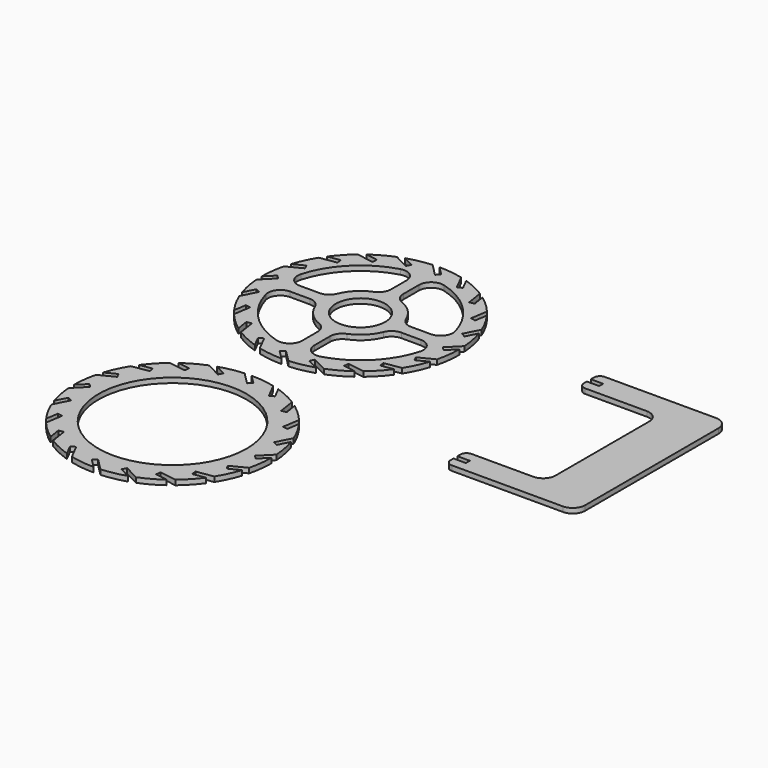
from build123d import *

# Parameters (mm, degrees)
F0_R     = 20
F1_DEPTH = 4
F0_R_2   = 60


# Not quite as in the source:
# - ends of sketch curves that miss each other by under 0.0002 mm in the source are joined


with BuildPart() as f1:
    # F0 (on Top) → F1 (new body)
    with BuildSketch(Plane.XY):
        with BuildLine():
            ThreePointArc((-98.2949099027, 172.7183773881), (-107.951775958, 174.5185802967), (-117.756472, 175.121679))
            Line((-117.756472, 175.121679), (-110.685404, 168.050611))
            Line((-110.685404, 168.050611), (-113.513831, 165.222184))
            Line((-113.513831, 165.222184), (-123.226125, 174.934478))
            ThreePointArc((-123.226125, 174.934478), (-132.9666439698, 173.6624370091), (-142.4778320463, 171.2062001424))
            Line((-142.4778320463, 171.2062001424), (-133.567766, 166.666295))
            Line((-133.567766, 166.666295), (-135.383728, 163.102269))
            Line((-135.383728, 163.102269), (-147.621933, 169.337946))
            ThreePointArc((-147.621933, 169.337946), (-156.4926341286, 165.1181769356), (-164.779292, 159.843038))
            Line((-164.779292, 159.843038), (-154.902409, 158.278694))
            Line((-154.902409, 158.278694), (-155.528147, 154.32794))
            Line((-155.528147, 154.32794), (-169.094301, 156.476608))
            ThreePointArc((-169.094301, 156.476608), (-176.2268590711, 149.7221719992), (-182.4778317927, 142.1444988494))
            Line((-182.4778317927, 142.1444988494), (-172.600948, 143.708844))
            Line((-172.600948, 143.708844), (-171.97521, 139.75809))
            Line((-171.97521, 139.75809), (-185.541364, 137.609423))
            ThreePointArc((-185.541364, 137.609423), (-190.2375947091, 128.9814907365), (-193.8409934363, 119.8430381417))
            Line((-193.8409934363, 119.8430381417), (-184.930928, 124.382943))
            Line((-184.930928, 124.382943), (-183.114966, 120.818917))
            Line((-183.114966, 120.818917), (-195.35317, 114.583241))
            ThreePointArc((-195.35317, 114.583241), (-197.1533732967, 104.926375042), (-197.756472, 95.121679))
            Line((-197.756472, 95.121679), (-190.685404, 102.192747))
            Line((-190.685404, 102.192747), (-187.856977, 99.36432))
            Line((-187.856977, 99.36432), (-197.569271, 89.652026))
            ThreePointArc((-197.569271, 89.652026), (-196.2972300091, 79.9115070302), (-193.8409931424, 70.4003189537))
            Line((-193.8409931424, 70.4003189537), (-189.301088, 79.310385))
            Line((-189.301088, 79.310385), (-185.737062, 77.494423))
            Line((-185.737062, 77.494423), (-191.972739, 65.256218))
            ThreePointArc((-191.972739, 65.256218), (-187.7529701762, 56.3855170442), (-182.4778317927, 48.0988591506))
            Line((-182.4778317927, 48.0988591506), (-180.913487, 57.975742))
            Line((-180.913487, 57.975742), (-176.962734, 57.350004))
            Line((-176.962734, 57.350004), (-179.111401, 43.78385))
            ThreePointArc((-179.111401, 43.78385), (-172.3569649992, 36.6512919289), (-164.7792918494, 30.4003192073))
            Line((-164.7792918494, 30.4003192073), (-166.343637, 40.277203))
            Line((-166.343637, 40.277203), (-162.392883, 40.902941))
            Line((-162.392883, 40.902941), (-160.244216, 27.336787))
            ThreePointArc((-160.244216, 27.336787), (-151.6162841674, 22.6405564922), (-142.4778320463, 19.0371578576))
            Line((-142.4778320463, 19.0371578576), (-147.017737, 27.947223))
            Line((-147.017737, 27.947223), (-143.45371, 29.763185))
            Line((-143.45371, 29.763185), (-137.218034, 17.52498))
            ThreePointArc((-137.218034, 17.52498), (-127.5611679213, 15.7247776884), (-117.756472, 15.121679))
            Line((-117.756472, 15.121679), (-124.82754, 22.192747))
            Line((-124.82754, 22.192747), (-121.999113, 25.021174))
            Line((-121.999113, 25.021174), (-112.286819, 15.30888))
            ThreePointArc((-112.286819, 15.30888), (-102.5463000302, 16.5809209909), (-93.0351119537, 19.0371578576))
            Line((-93.0351119537, 19.0371578576), (-101.945178, 23.577063))
            Line((-101.945178, 23.577063), (-100.129216, 27.141089))
            Line((-100.129216, 27.141089), (-87.891011, 20.905412))
            ThreePointArc((-87.891011, 20.905412), (-79.0203100442, 25.1251808238), (-70.7336521506, 30.4003192073))
            Line((-70.7336521506, 30.4003192073), (-80.610535, 31.964664))
            Line((-80.610535, 31.964664), (-79.984797, 35.915417))
            Line((-79.984797, 35.915417), (-66.418643, 33.76675))
            ThreePointArc((-66.418643, 33.76675), (-59.2860849289, 40.5211860008), (-53.0351122073, 48.0988591506))
            Line((-53.0351122073, 48.0988591506), (-62.911996, 46.534514))
            Line((-62.911996, 46.534514), (-63.537734, 50.485267))
            Line((-63.537734, 50.485267), (-49.97158, 52.633935))
            ThreePointArc((-49.97158, 52.633935), (-45.2753494922, 61.2618668326), (-41.6719508576, 70.4003189537))
            Line((-41.6719508576, 70.4003189537), (-50.582016, 65.860414))
            Line((-50.582016, 65.860414), (-52.397978, 69.42444))
            Line((-52.397978, 69.42444), (-40.159774, 75.660117))
            ThreePointArc((-40.159774, 75.660117), (-38.3595707033, 85.316982958), (-37.756472, 95.121679))
            Line((-37.756472, 95.121679), (-44.82754, 88.050611))
            Line((-44.82754, 88.050611), (-47.655967, 90.879038))
            Line((-47.655967, 90.879038), (-37.943673, 100.591332))
            ThreePointArc((-37.943673, 100.591332), (-39.2157139005, 110.3318505029), (-41.6719505637, 119.8430381417))
            Line((-41.6719505637, 119.8430381417), (-46.211856, 110.932973))
            Line((-46.211856, 110.932973), (-49.775882, 112.748935))
            Line((-49.775882, 112.748935), (-43.540205, 124.98714))
            ThreePointArc((-43.540205, 124.98714), (-47.7599738238, 133.8578409558), (-53.0351122073, 142.1444988494))
            Line((-53.0351122073, 142.1444988494), (-54.599457, 132.267616))
            Line((-54.599457, 132.267616), (-58.55021, 132.893354))
            Line((-58.55021, 132.893354), (-56.401543, 146.459508))
            ThreePointArc((-56.401543, 146.459508), (-63.155978786, 153.5920658705), (-70.7336516751, 159.8430384472))
            Line((-70.7336516751, 159.8430384472), (-69.169307, 149.966155))
            Line((-69.169307, 149.966155), (-73.120061, 149.340417))
            Line((-73.120061, 149.340417), (-75.268728, 162.906571))
            ThreePointArc((-75.268728, 162.906571), (-83.8966598326, 167.6028015078), (-93.0351119537, 171.2062001424))
            Line((-93.0351119537, 171.2062001424), (-88.495207, 162.296135))
            Line((-88.495207, 162.296135), (-92.059234, 160.480173))
            Line((-92.059234, 160.480173), (-98.2949099027, 172.7183773881))
        make_face()
        with BuildLine():
            Line((-170.673856, 90.129798), (-154.840804, 90.129798))
            ThreePointArc((-154.840804, 90.129798), (-149.2497262903, 88.420747888), (-145.5697349779, 83.8777680089))
            ThreePointArc((-145.5697349779, 83.8777680089), (-138.9697319753, 73.9084751041), (-129.0004390268, 67.3084719338))
            ThreePointArc((-129.0004390268, 67.3084719338), (-124.4574598529, 63.6284803253), (-122.74841, 58.037403))
            Line((-122.74841, 58.037403), (-122.74841, 42.204352))
            ThreePointArc((-122.74841, 42.204352), (-126.7175709587, 34.2275744265), (-135.4742060915, 32.5830196771))
            ThreePointArc((-135.4742060915, 32.5830196771), (-163.718469437, 49.1597378827), (-180.2951881241, 77.4040009648))
            ThreePointArc((-180.2951881241, 77.4040009648), (-178.6506338636, 86.1606366576), (-170.673856, 90.129798))
        make_face(mode=Mode.SUBTRACT)
        with BuildLine():
            Line((-112.764647, 42.204352), (-112.764647, 58.037403))
            ThreePointArc((-112.764647, 58.037403), (-111.0555971471, 63.6284803253), (-106.5126178685, 67.3084716746))
            ThreePointArc((-106.5126178685, 67.3084716746), (-96.5433255644, 73.9084755644), (-89.9433222812, 83.8777681137))
            ThreePointArc((-89.9433222812, 83.8777681137), (-86.2633307097, 88.420747888), (-80.672253, 90.129798))
            Line((-80.672253, 90.129798), (-64.839202, 90.129798))
            ThreePointArc((-64.839202, 90.129798), (-56.8624242186, 86.1606367663), (-55.2178698651, 77.4040012451))
            ThreePointArc((-55.2178698651, 77.4040012451), (-71.7945881265, 49.1597383192), (-100.0388509648, 32.5830198759))
            ThreePointArc((-100.0388509648, 32.5830198759), (-108.7954860413, 34.2275744265), (-112.764647, 42.204352))
        make_face(mode=Mode.SUBTRACT)
        with Locations((-117.756529, 95.121679)):
            Circle(F0_R, mode=Mode.SUBTRACT)
        with BuildLine():
            ThreePointArc((-145.5697349779, 106.3655899911), (-149.2497262903, 101.822610112), (-154.840804, 100.11356))
            Line((-154.840804, 100.11356), (-170.673856, 100.11356))
            ThreePointArc((-170.673856, 100.11356), (-178.6506338636, 104.0827213424), (-180.2951880606, 112.8393570172))
            ThreePointArc((-180.2951880606, 112.8393570172), (-163.718469437, 141.0836201173), (-135.4742061095, 157.6603383864))
            ThreePointArc((-135.4742061095, 157.6603383864), (-126.7175709587, 156.0157835735), (-122.74841, 148.039006))
            Line((-122.74841, 148.039006), (-122.74841, 132.205954))
            ThreePointArc((-122.74841, 132.205954), (-124.4574597481, 126.61487683), (-129.0004387841, 122.9348854659))
            ThreePointArc((-129.0004387841, 122.9348854659), (-138.9697319753, 116.3348828959), (-145.5697349779, 106.3655899911))
        make_face(mode=Mode.SUBTRACT)
        with BuildLine():
            Line((-64.839202, 100.11356), (-80.672253, 100.11356))
            ThreePointArc((-80.672253, 100.11356), (-86.2633307097, 101.822610112), (-89.9433220221, 106.3655899911))
            ThreePointArc((-89.9433220221, 106.3655899911), (-96.5433255644, 116.3348824356), (-106.5126181137, 122.9348857188))
            ThreePointArc((-106.5126181137, 122.9348857188), (-111.0555972519, 126.61487683), (-112.764647, 132.205954))
            Line((-112.764647, 132.205954), (-112.764647, 148.039006))
            ThreePointArc((-112.764647, 148.039006), (-108.7954860413, 156.0157835735), (-100.0388509085, 157.6603383229))
            ThreePointArc((-100.0388509085, 157.6603383229), (-71.7945881265, 141.0836196808), (-55.2178698016, 112.8393567729))
            ThreePointArc((-55.2178698016, 112.8393567729), (-56.8624242186, 104.0827212337), (-64.839202, 100.11356))
        make_face(mode=Mode.SUBTRACT)
    extrude(amount=F1_DEPTH)


with BuildPart() as f1b:
    # F0 (on Top) → F1, piece 2 (new body)
    with BuildSketch(Plane.XY):
        with BuildLine():
            ThreePointArc((-98.2949099027, -17.5249796119), (-107.951775958, -15.7247767033), (-117.756472, -15.121678))
            Line((-117.756472, -15.121678), (-110.685404, -22.192746))
            Line((-110.685404, -22.192746), (-113.513831, -25.021173))
            Line((-113.513831, -25.021173), (-123.226125, -15.308879))
            ThreePointArc((-123.226125, -15.308879), (-132.9666439698, -16.5809199909), (-142.4778320463, -19.0371568576))
            Line((-142.4778320463, -19.0371568576), (-133.567766, -23.577062))
            Line((-133.567766, -23.577062), (-135.383728, -27.141088))
            Line((-135.383728, -27.141088), (-147.621933, -20.905411))
            ThreePointArc((-147.621933, -20.905411), (-156.4926340905, -25.1251795775), (-164.779292, -30.400318))
            Line((-164.779292, -30.400318), (-154.902409, -31.964663))
            Line((-154.902409, -31.964663), (-155.528147, -35.915416))
            Line((-155.528147, -35.915416), (-169.094301, -33.766749))
            ThreePointArc((-169.094301, -33.766749), (-176.2268590711, -40.5211850008), (-182.4778317927, -48.0988581506))
            Line((-182.4778317927, -48.0988581506), (-172.600948, -46.534513))
            Line((-172.600948, -46.534513), (-171.97521, -50.485267))
            Line((-171.97521, -50.485267), (-185.541364, -52.633934))
            ThreePointArc((-185.541364, -52.633934), (-190.2375945078, -61.2618658326), (-193.8409931424, -70.4003179537))
            Line((-193.8409931424, -70.4003179537), (-184.930928, -65.860413))
            Line((-184.930928, -65.860413), (-183.114966, -69.42444))
            Line((-183.114966, -69.42444), (-195.35317, -75.660116))
            ThreePointArc((-195.35317, -75.660116), (-197.1533732967, -85.316981958), (-197.756472, -95.121678))
            Line((-197.756472, -95.121678), (-190.685404, -88.05061))
            Line((-190.685404, -88.05061), (-187.856977, -90.879037))
            Line((-187.856977, -90.879037), (-197.569271, -100.591331))
            ThreePointArc((-197.569271, -100.591331), (-196.2972300091, -110.3318499698), (-193.8409931424, -119.8430380463))
            Line((-193.8409931424, -119.8430380463), (-189.301088, -110.932972))
            Line((-189.301088, -110.932972), (-185.737062, -112.748934))
            Line((-185.737062, -112.748934), (-191.972739, -124.987139))
            ThreePointArc((-191.972739, -124.987139), (-187.7529701762, -133.8578399558), (-182.4778317927, -142.1444978494))
            Line((-182.4778317927, -142.1444978494), (-180.913487, -132.267615))
            Line((-180.913487, -132.267615), (-176.962734, -132.893353))
            Line((-176.962734, -132.893353), (-179.111401, -146.459507))
            ThreePointArc((-179.111401, -146.459507), (-172.3569649992, -153.5920650711), (-164.7792918494, -159.8430377927))
            Line((-164.7792918494, -159.8430377927), (-166.343637, -149.966154))
            Line((-166.343637, -149.966154), (-162.392883, -149.340416))
            Line((-162.392883, -149.340416), (-160.244216, -162.90657))
            ThreePointArc((-160.244216, -162.90657), (-151.6162841674, -167.6028005078), (-142.4778320463, -171.2061991424))
            Line((-142.4778320463, -171.2061991424), (-147.017737, -162.296134))
            Line((-147.017737, -162.296134), (-143.45371, -160.480172))
            Line((-143.45371, -160.480172), (-137.218034, -172.718376))
            ThreePointArc((-137.218034, -172.718376), (-127.561168042, -174.5185792967), (-117.756472, -175.121678))
            Line((-117.756472, -175.121678), (-124.82754, -168.05061))
            Line((-124.82754, -168.05061), (-121.999113, -165.222183))
            Line((-121.999113, -165.222183), (-112.286819, -174.934477))
            ThreePointArc((-112.286819, -174.934477), (-102.5463000302, -173.6624360091), (-93.0351119537, -171.2061991424))
            Line((-93.0351119537, -171.2061991424), (-101.945178, -166.666294))
            Line((-101.945178, -166.666294), (-100.129216, -163.102268))
            Line((-100.129216, -163.102268), (-87.891011, -169.337945))
            ThreePointArc((-87.891011, -169.337945), (-79.0203100442, -165.1181761762), (-70.7336521506, -159.8430377927))
            Line((-70.7336521506, -159.8430377927), (-80.610535, -158.278693))
            Line((-80.610535, -158.278693), (-79.984797, -154.32794))
            Line((-79.984797, -154.32794), (-66.418643, -156.476607))
            ThreePointArc((-66.418643, -156.476607), (-59.2860849289, -149.7221709992), (-53.0351122073, -142.1444978494))
            Line((-53.0351122073, -142.1444978494), (-62.911996, -143.708843))
            Line((-62.911996, -143.708843), (-63.537734, -139.758089))
            Line((-63.537734, -139.758089), (-49.97158, -137.609422))
            ThreePointArc((-49.97158, -137.609422), (-45.2753494922, -128.9814901674), (-41.6719508576, -119.8430380463))
            Line((-41.6719508576, -119.8430380463), (-50.582016, -124.382943))
            Line((-50.582016, -124.382943), (-52.397978, -120.818916))
            Line((-52.397978, -120.818916), (-40.159774, -114.58324))
            ThreePointArc((-40.159774, -114.58324), (-38.3595707033, -104.926374042), (-37.756472, -95.121678))
            Line((-37.756472, -95.121678), (-44.82754, -102.192746))
            Line((-44.82754, -102.192746), (-47.655967, -99.364319))
            Line((-47.655967, -99.364319), (-37.943673, -89.652025))
            ThreePointArc((-37.943673, -89.652025), (-39.2157139909, -79.9115060302), (-41.6719508576, -70.4003179537))
            Line((-41.6719508576, -70.4003179537), (-46.211856, -79.310384))
            Line((-46.211856, -79.310384), (-49.775882, -77.494422))
            Line((-49.775882, -77.494422), (-43.540205, -65.256217))
            ThreePointArc((-43.540205, -65.256217), (-47.7599738238, -56.3855160442), (-53.0351122073, -48.0988581506))
            Line((-53.0351122073, -48.0988581506), (-54.599457, -57.975741))
            Line((-54.599457, -57.975741), (-58.55021, -57.350003))
            Line((-58.55021, -57.350003), (-56.401543, -43.783849))
            ThreePointArc((-56.401543, -43.783849), (-63.1559790008, -36.6512909289), (-70.7336521506, -30.4003182073))
            Line((-70.7336521506, -30.4003182073), (-69.169307, -40.277202))
            Line((-69.169307, -40.277202), (-73.120061, -40.90294))
            Line((-73.120061, -40.90294), (-75.268728, -27.336786))
            ThreePointArc((-75.268728, -27.336786), (-83.8966598326, -22.6405554922), (-93.0351119537, -19.0371568576))
            Line((-93.0351119537, -19.0371568576), (-88.495207, -27.947222))
            Line((-88.495207, -27.947222), (-92.059234, -29.763184))
            Line((-92.059234, -29.763184), (-98.2949099027, -17.5249796119))
        make_face()
        with Locations((-117.756472, -95.121678)):
            Circle(F0_R_2, mode=Mode.SUBTRACT)
    extrude(amount=F1_DEPTH)


with BuildPart() as f1c:
    # F0 (on Top) → F1, piece 3 (new body)
    with BuildSketch(Plane.XY):
        with BuildLine():
            Line((147.756471, 123.123724), (57.756471, 123.123724))
            ThreePointArc((57.756471, 123.123724), (54.2209370941, 121.6592579059), (52.756471, 118.123724))
            Line((52.756471, 118.123724), (52.756471, 115.123724))
            Line((52.756471, 115.123724), (62.756471, 115.123724))
            Line((62.756471, 115.123724), (62.756471, 111.123724))
            Line((62.756471, 111.123724), (52.756471, 111.123724))
            Line((52.756471, 111.123724), (52.756471, 108.123724))
            ThreePointArc((52.756471, 108.123724), (54.2209370941, 104.5881900941), (57.756471, 103.123724))
            Line((57.756471, 103.123724), (107.756471, 103.123724))
            ThreePointArc((107.756471, 103.123724), (114.8275388119, 100.1947918119), (117.756471, 93.123724))
            Line((117.756471, 93.123724), (117.756471, -1.876276))
            ThreePointArc((117.756471, -1.876276), (114.8275388119, -8.9473438119), (107.756471, -11.876276))
            Line((107.756471, -11.876276), (57.756471, -11.876276))
            ThreePointArc((57.756471, -11.876276), (54.2209370941, -13.3407420941), (52.756471, -16.876276))
            Line((52.756471, -16.876276), (52.756471, -19.876276))
            Line((52.756471, -19.876276), (62.756471, -19.876276))
            Line((62.756471, -19.876276), (62.756471, -23.876276))
            Line((62.756471, -23.876276), (52.756471, -23.876276))
            Line((52.756471, -23.876276), (52.756471, -26.876276))
            ThreePointArc((52.756471, -26.876276), (54.2209370941, -30.4118099059), (57.756471, -31.876276))
            Line((57.756471, -31.876276), (147.756471, -31.876276))
            ThreePointArc((147.756471, -31.876276), (154.8275388119, -28.9473438119), (157.756471, -21.876276))
            Line((157.756471, -21.876276), (157.756471, 113.123724))
            ThreePointArc((157.756471, 113.123724), (154.8275388119, 120.1947918119), (147.756471, 123.123724))
        make_face()
    extrude(amount=F1_DEPTH)


solid = Compound([f1.part, f1b.part, f1c.part])
